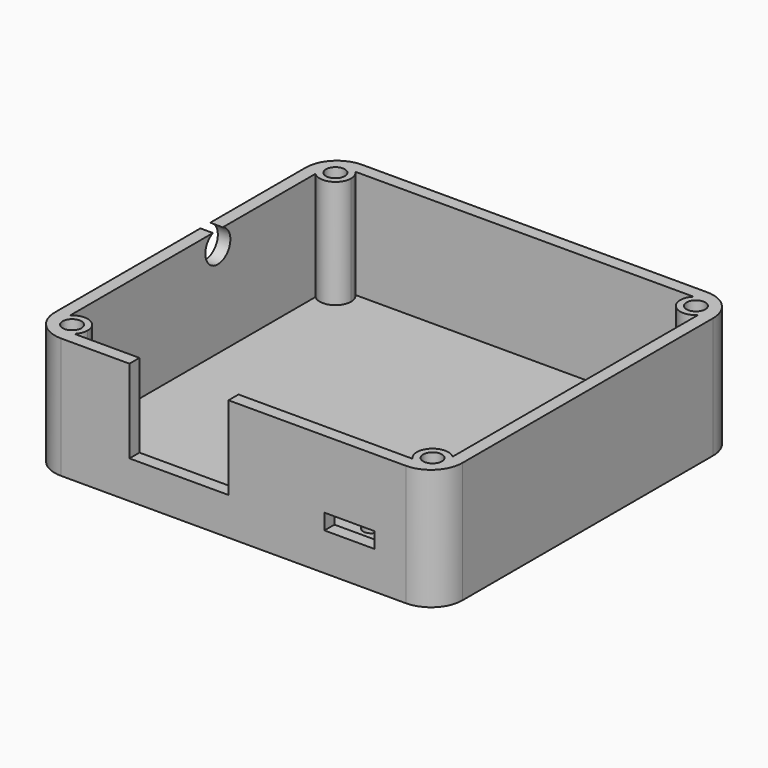
from build123d import *

# Parameters (mm, degrees)
F0_W      = 65
F0_H      = 60
F1_DEPTH  = 17.3
F3_START  = 25
F2_W      = 15.8
F2_H      = 13.3
F3_DEPTH  = 2.5
F5_D      = 5
F5_DEPTH  = 32.501
F2_W_2    = 8
F2_H_2    = 2.5
F6_DEPTH  = 30
F0_R      = 1.25
F7_DEPTH  = 2
F8_DEPTH  = 5
F9_DEPTH  = 17.3
F10_D     = 3
F10_DEPTH = 22
F10_TIP   = 0.9012909285
F11_DEPTH = 30
F12_R     = 5


# Not quite as in the source:
# - a feature names something its author has since deleted; it is built from what else it names


with BuildPart() as f1:
    # F0 (on Top) → F1 (new body)
    with BuildSketch(Plane.XY):
        Rectangle(F0_W, F0_H)
        with BuildLine():
            ThreePointArc((-30.5, 24.4646428929), (-30.517766953, 28.017766953), (-26.9646428929, 28))
            Line((-26.9646428929, 28), (26.9646428929, 28))
            ThreePointArc((26.9646428929, 28), (29.6951474044, 28.5644537982), (31.25, 26.25))
            ThreePointArc((31.25, 26.25), (31.0548861143, 25.2817541634), (30.5, 24.4646428929))
            Line((30.5, 24.4646428929), (30.5, -24.4646428929))
            ThreePointArc((30.5, -24.4646428929), (31.0548861143, -25.2817541634), (31.25, -26.25))
            ThreePointArc((31.25, -26.25), (29.6951474044, -28.5644537982), (26.9646428929, -28))
            Line((26.9646428929, -28), (-26.9646428929, -28))
            ThreePointArc((-26.9646428929, -28), (-30.517766953, -28.017766953), (-30.5, -24.4646428929))
            Line((-30.5, -24.4646428929), (-30.5, 24.4646428929))
        make_face(mode=Mode.SUBTRACT)
    extrude(amount=F1_DEPTH)

    # F2 (on Front) → F3 (cut)
    with BuildSketch(Plane.XZ.offset(F3_START)):
        with Locations((-8.7, 10.65)):
            Rectangle(F2_W, F2_H)
    extrude(amount=F3_DEPTH, mode=Mode.SUBTRACT)

    # F5 (through all, one way)
    with BuildSketch(Plane.YZ):
        with Locations((5, 15)):
            Circle(F5_D / 2)
    extrude(amount=-F5_DEPTH, mode=Mode.SUBTRACT)

    # F2 (on Front) → F6 (cut)
    with BuildSketch(Plane.XZ):
        with Locations((18.5, 5.25)):
            Rectangle(F2_W_2, F2_H_2)
    extrude(amount=F6_DEPTH, mode=Mode.SUBTRACT)

    # F0 (on Top) → F7 (join)
    with BuildSketch(Plane.XY):
        Rectangle(F0_W, F0_H)
        with BuildLine():
            ThreePointArc((-30.5, 24.4646428929), (-30.517766953, 28.017766953), (-26.9646428929, 28))
            Line((-26.9646428929, 28), (26.9646428929, 28))
            ThreePointArc((26.9646428929, 28), (29.6951474044, 28.5644537982), (31.25, 26.25))
            ThreePointArc((31.25, 26.25), (31.0548861143, 25.2817541634), (30.5, 24.4646428929))
            Line((30.5, 24.4646428929), (30.5, -24.4646428929))
            ThreePointArc((30.5, -24.4646428929), (31.0548861143, -25.2817541634), (31.25, -26.25))
            ThreePointArc((31.25, -26.25), (29.6951474044, -28.5644537982), (26.9646428929, -28))
            Line((26.9646428929, -28), (-26.9646428929, -28))
            ThreePointArc((-26.9646428929, -28), (-30.517766953, -28.017766953), (-30.5, -24.4646428929))
            Line((-30.5, -24.4646428929), (-30.5, 24.4646428929))
        make_face(mode=Mode.SUBTRACT)
        with BuildLine():
            Line((26.9646428929, 28), (-26.9646428929, 28))
            ThreePointArc((-26.9646428929, 28), (-26.4355462018, 27.1951474044), (-26.25, 26.25))
            ThreePointArc((-26.25, 26.25), (-27.7817541634, 23.9451138857), (-30.5, 24.4646428929))
            Line((-30.5, 24.4646428929), (-30.5, -24.4646428929))
            ThreePointArc((-30.5, -24.4646428929), (-27.7817541634, -23.9451138857), (-26.25, -26.25))
            ThreePointArc((-26.25, -26.25), (-26.4355462018, -27.1951474044), (-26.9646428929, -28))
            Line((-26.9646428929, -28), (26.9646428929, -28))
            ThreePointArc((26.9646428929, -28), (26.982233047, -24.482233047), (30.5, -24.4646428929))
            Line((30.5, -24.4646428929), (30.5, 24.4646428929))
            ThreePointArc((30.5, 24.4646428929), (26.982233047, 24.482233047), (26.9646428929, 28))
        make_face()
        with Locations((-22.5, -24)):
            Circle(F0_R, mode=Mode.SUBTRACT)
        with Locations((4.5, -24)):
            Circle(F0_R, mode=Mode.SUBTRACT)
        with Locations((13.95, -20)):
            Circle(F0_R, mode=Mode.SUBTRACT)
        with Locations((22.5, -20)):
            Circle(F0_R, mode=Mode.SUBTRACT)
        with BuildLine():
            Line((-26.9646428929, 28), (-30.5, 28))
            Line((-30.5, 28), (-30.5, 24.4646428929))
            ThreePointArc((-30.5, 24.4646428929), (-27.7817541634, 23.9451138857), (-26.25, 26.25))
            ThreePointArc((-26.25, 26.25), (-26.4355462018, 27.1951474044), (-26.9646428929, 28))
        make_face()
        with BuildLine():
            Line((30.5, 28), (26.9646428929, 28))
            ThreePointArc((26.9646428929, 28), (26.982233047, 24.482233047), (30.5, 24.4646428929))
            Line((30.5, 24.4646428929), (30.5, 28))
        make_face()
        with BuildLine():
            ThreePointArc((-26.25, -26.25), (-27.7817541634, -23.9451138857), (-30.5, -24.4646428929))
            Line((-30.5, -24.4646428929), (-30.5, -28))
            Line((-30.5, -28), (-26.9646428929, -28))
            ThreePointArc((-26.9646428929, -28), (-26.4355462018, -27.1951474044), (-26.25, -26.25))
        make_face()
        with BuildLine():
            Line((30.5, -28), (30.5, -24.4646428929))
            ThreePointArc((30.5, -24.4646428929), (26.982233047, -24.482233047), (26.9646428929, -28))
            Line((26.9646428929, -28), (30.5, -28))
        make_face()
        with Locations((22.5, -20)):
            Circle(F0_R)
        with Locations((13.95, -20)):
            Circle(F0_R)
        with Locations((-22.5, -24)):
            Circle(F0_R)
        with Locations((4.5, -24)):
            Circle(F0_R)
        with BuildLine():
            Line((-30.5, 24.4646428929), (-30.5, 28))
            Line((-30.5, 28), (-26.9646428929, 28))
            ThreePointArc((-26.9646428929, 28), (-30.517766953, 28.017766953), (-30.5, 24.4646428929))
        make_face()
        with BuildLine():
            ThreePointArc((31.25, 26.25), (29.6951474044, 28.5644537982), (26.9646428929, 28))
            Line((26.9646428929, 28), (30.5, 28))
            Line((30.5, 28), (30.5, 24.4646428929))
            ThreePointArc((30.5, 24.4646428929), (31.0548861143, 25.2817541634), (31.25, 26.25))
        make_face()
        with BuildLine():
            Line((-30.5, -28), (-30.5, -24.4646428929))
            ThreePointArc((-30.5, -24.4646428929), (-30.517766953, -28.017766953), (-26.9646428929, -28))
            Line((-26.9646428929, -28), (-30.5, -28))
        make_face()
        with BuildLine():
            ThreePointArc((31.25, -26.25), (31.0548861143, -25.2817541634), (30.5, -24.4646428929))
            Line((30.5, -24.4646428929), (30.5, -28))
            Line((30.5, -28), (26.9646428929, -28))
            ThreePointArc((26.9646428929, -28), (29.6951474044, -28.5644537982), (31.25, -26.25))
        make_face()
    extrude(amount=-F7_DEPTH)

    # F0 (on Top) → F8 (join)
    with BuildSketch(Plane.XY):
        with Locations((22.5, -20)):
            Circle(F0_R)
        with Locations((13.95, -20)):
            Circle(F0_R)
        with Locations((-22.5, -24)):
            Circle(F0_R)
        with Locations((4.5, -24)):
            Circle(F0_R)
    extrude(amount=F8_DEPTH)

    # F0 (on Top) → F9 (join)
    with BuildSketch(Plane.XY):
        with BuildLine():
            Line((30.5, -28), (30.5, -24.4646428929))
            ThreePointArc((30.5, -24.4646428929), (26.982233047, -24.482233047), (26.9646428929, -28))
            Line((26.9646428929, -28), (30.5, -28))
        make_face()
        with BuildLine():
            ThreePointArc((31.25, -26.25), (31.0548861143, -25.2817541634), (30.5, -24.4646428929))
            Line((30.5, -24.4646428929), (30.5, -28))
            Line((30.5, -28), (26.9646428929, -28))
            ThreePointArc((26.9646428929, -28), (29.6951474044, -28.5644537982), (31.25, -26.25))
        make_face()
        with BuildLine():
            ThreePointArc((31.25, 26.25), (29.6951474044, 28.5644537982), (26.9646428929, 28))
            Line((26.9646428929, 28), (30.5, 28))
            Line((30.5, 28), (30.5, 24.4646428929))
            ThreePointArc((30.5, 24.4646428929), (31.0548861143, 25.2817541634), (31.25, 26.25))
        make_face()
        with BuildLine():
            Line((30.5, 28), (26.9646428929, 28))
            ThreePointArc((26.9646428929, 28), (26.982233047, 24.482233047), (30.5, 24.4646428929))
            Line((30.5, 24.4646428929), (30.5, 28))
        make_face()
        with BuildLine():
            Line((-26.9646428929, 28), (-30.5, 28))
            Line((-30.5, 28), (-30.5, 24.4646428929))
            ThreePointArc((-30.5, 24.4646428929), (-27.7817541634, 23.9451138857), (-26.25, 26.25))
            ThreePointArc((-26.25, 26.25), (-26.4355462018, 27.1951474044), (-26.9646428929, 28))
        make_face()
        with BuildLine():
            Line((-30.5, 24.4646428929), (-30.5, 28))
            Line((-30.5, 28), (-26.9646428929, 28))
            ThreePointArc((-26.9646428929, 28), (-30.517766953, 28.017766953), (-30.5, 24.4646428929))
        make_face()
        with BuildLine():
            Line((-30.5, -28), (-30.5, -24.4646428929))
            ThreePointArc((-30.5, -24.4646428929), (-30.517766953, -28.017766953), (-26.9646428929, -28))
            Line((-26.9646428929, -28), (-30.5, -28))
        make_face()
        with BuildLine():
            ThreePointArc((-26.25, -26.25), (-27.7817541634, -23.9451138857), (-30.5, -24.4646428929))
            Line((-30.5, -24.4646428929), (-30.5, -28))
            Line((-30.5, -28), (-26.9646428929, -28))
            ThreePointArc((-26.9646428929, -28), (-26.4355462018, -27.1951474044), (-26.25, -26.25))
        make_face()
    extrude(amount=F9_DEPTH)

    # F10 (one way)
    with BuildSketch(Plane(origin=(0, 0, 0), x_dir=(1, 0, 0), z_dir=(0, 0, -1))):
        with Locations((-28.75, -26.25), (28.75, -26.25), (28.75, 26.25), (-28.75, 26.25)):
            Circle(F10_D / 2)
    extrude(amount=-F10_DEPTH, mode=Mode.SUBTRACT)
    with Locations(Plane(origin=(0, 0, 0), x_dir=(1, 0, 0), z_dir=(0, 0, -1))):
        with Locations((-28.75, -26.25), (28.75, -26.25), (28.75, 26.25), (-28.75, 26.25)):
            with Locations((0, 0, -(F10_DEPTH + F10_TIP / 2))):  # 118° drill point
                Cone(0, F10_D / 2, F10_TIP, mode=Mode.SUBTRACT)

    # F2 (on Front) → F11 (cut)
    with BuildSketch(Plane.XZ):
        with Locations((-8.7, 10.65)):
            Rectangle(F2_W, F2_H)
    extrude(amount=F11_DEPTH, mode=Mode.SUBTRACT)

    # F12
    f12_edges = [f1.edges().sort_by_distance(p)[0] for p in [
        (32.5, -30, 7.65),
        (32.5, 30, 7.65),
        (-32.5, 30, 7.65),
        (-32.5, -30, 7.65),
    ]]
    fillet(f12_edges, radius=F12_R)


solid = f1.part
